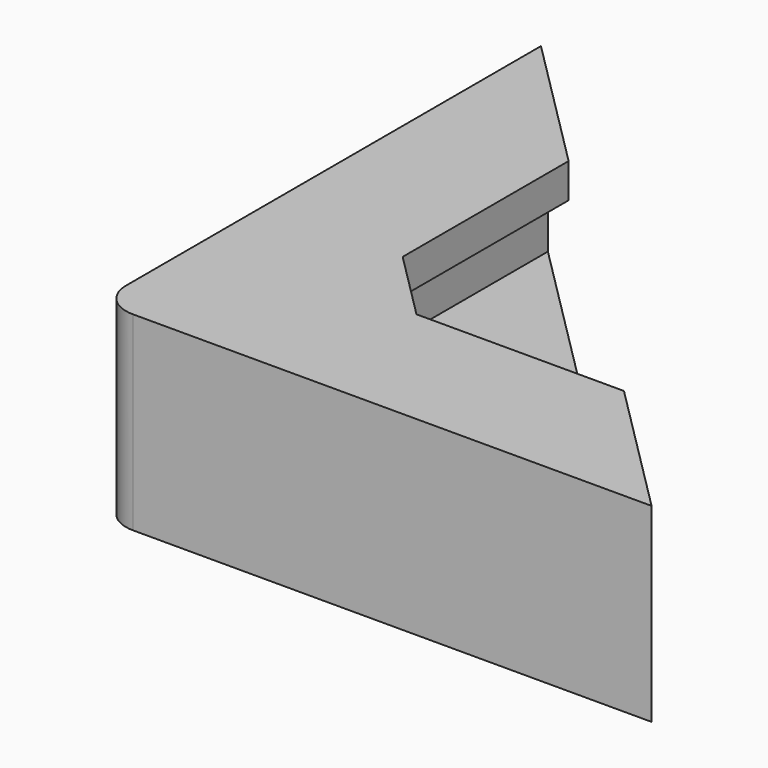
from build123d import *

# Parameters (mm, degrees)
F1_DEPTH = 2
F3_DEPTH = 25
F5_DEPTH = 7
F7_DEPTH = 2
F8_SIZE2 = 0.5773502692
F8_SIZE  = 1
F9_R     = 2


with BuildPart() as f1:
    # F0 (on Top) → F1 (new body)
    with BuildSketch(Plane.XY):
        Polygon((0, 32), (0, 0), (32, 0), align=None)
    extrude(amount=F1_DEPTH)

    # F2 (on face) → F3 (cut)
    with BuildSketch(Plane.XY.offset(2)):
        with BuildLine():
            Line((11.0502525317, 20.9497474683), (7.1611652352, 17.0606601718))
            ThreePointArc((7.1611652352, 17.0606601718), (7.1611652352, 7.1611652352), (17.0606601718, 7.1611652352))
            Line((17.0606601718, 7.1611652352), (20.9497474683, 11.0502525317))
            Line((20.9497474683, 11.0502525317), (11.0502525317, 20.9497474683))
        make_face()
    extrude(amount=-F3_DEPTH, mode=Mode.SUBTRACT)

    # F4 (on face) → F5 (join)
    with BuildSketch(Plane.XY.offset(2)):
        Polygon((0, 32), (0, 0), (32, 0), (30, 2), (2, 2), (2, 30), align=None)
    extrude(amount=F5_DEPTH)

    # F6 (on face) → F7 (join)
    with BuildSketch(Plane.XY.offset(9)):
        Polygon((0, 32), (0, 0), (32, 0), (30, 2), (24, 8), (12, 8), (8, 12), (8, 24), (2, 30), align=None)
    extrude(amount=F7_DEPTH)

    # F8
    f8_edges = [f1.edges().sort_by_distance(p)[0] for p in [
        (10, 10, 9),
    ]]
    chamfer(f8_edges, length=F8_SIZE, length2=F8_SIZE2)

    # F9
    f9_edges = [f1.edges().sort_by_distance(p)[0] for p in [
        (0, 0, 5.5),
    ]]
    fillet(f9_edges, radius=F9_R)


solid = f1.part
